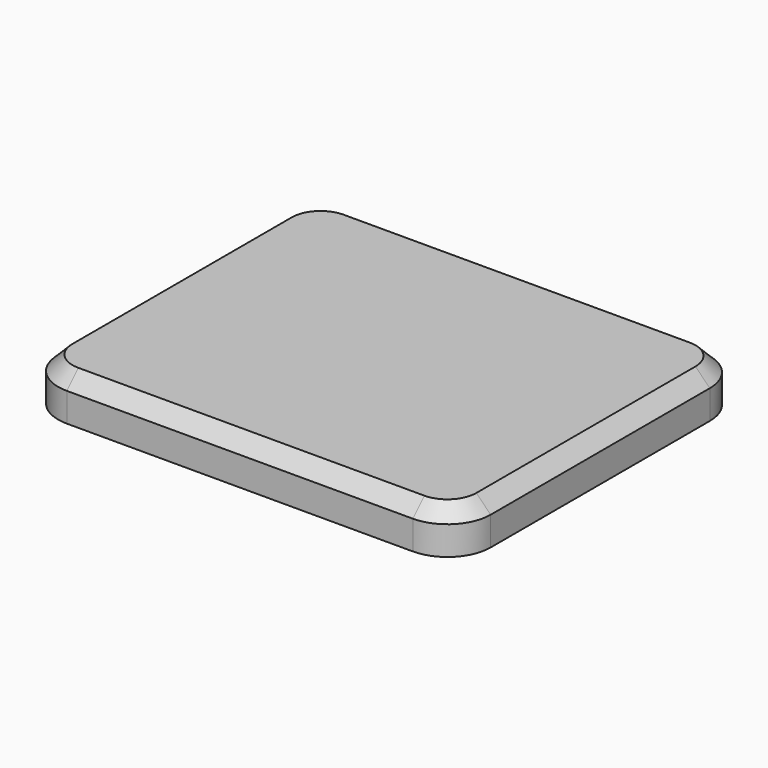
from build123d import *

# Parameters (mm, degrees)
F0_W     = 300
F0_H     = 250
F1_DEPTH = 30
F2_R     = 30
F3_SIZE2 = 10
F3_SIZE  = 10


with BuildPart() as f1:
    # F0 (on Top) → F1 (new body)
    with BuildSketch(Plane.XY):
        Rectangle(F0_W, F0_H)
    extrude(amount=F1_DEPTH)

    # F2
    f2_edges = [f1.edges().sort_by_distance(p)[0] for p in [
        (-150, -125, 15),
        (-150, 125, 15),
        (150, 125, 15),
        (150, -125, 15),
    ]]
    fillet(f2_edges, radius=F2_R)

    # F3
    f3_edges = [f1.edges().sort_by_distance(p)[0] for p in [
        (-150, 0, 30),
        (0, 125, 30),
        (150, 0, 30),
        (0, -125, 30),
        (141.213203, -116.213203, 30),
        (141.213203, 116.213203, 30),
        (-141.213203, -116.213203, 30),
        (-141.213203, 116.213203, 30),
    ]]
    chamfer(f3_edges, length=F3_SIZE, length2=F3_SIZE2)


solid = f1.part
